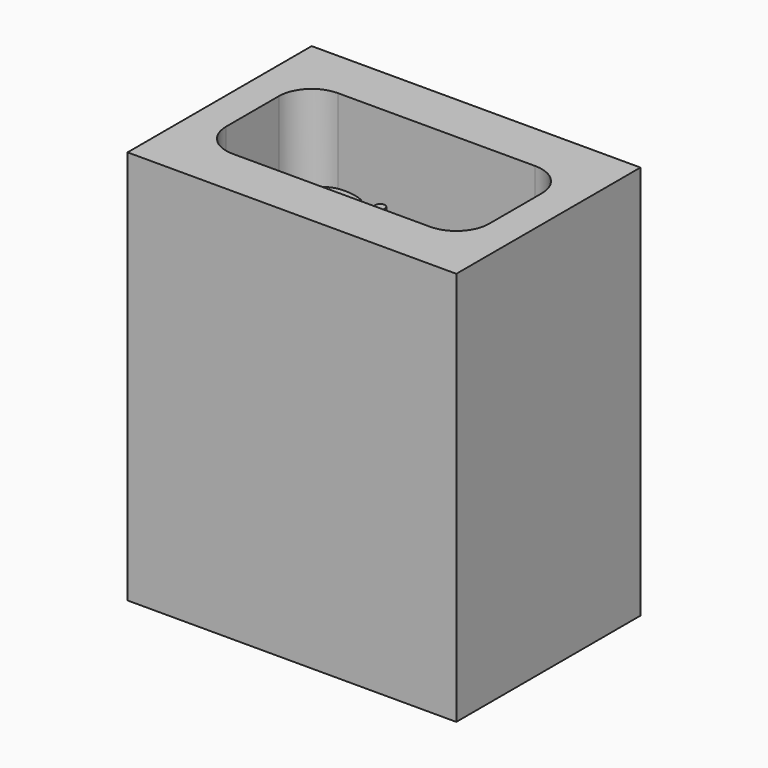
from build123d import *

# Parameters (mm, degrees)
F0_W         = 1000
F0_H         = 700
F1_DEPTH     = 1200
F3_DEPTH     = 300
F4_TEXT_SIZE = 300.7989973367
F5_DEPTH     = 100


# Not quite as in the source:
# - Text() gives the source's letters only with a copy of the font that has no kerning and outlines rounded to 1/6400 em; it was checked with that copy


with BuildPart() as f1:
    # F0 (on Top) → F1 (new body)
    with BuildSketch(Plane.XY):
        Rectangle(F0_W, F0_H)
    extrude(amount=F1_DEPTH)

    # F2 (on face) → F3 (cut)
    with BuildSketch(Plane.XY.offset(1200)):
        with BuildLine():
            Line((-300, -200), (300, -200))
            ThreePointArc((300, -200), (370.7106781187, -170.7106781187), (400, -100))
            Line((400, -100), (400, 100))
            ThreePointArc((400, 100), (370.7106781187, 170.7106781187), (300, 200))
            Line((300, 200), (-300, 200))
            ThreePointArc((-300, 200), (-370.7106781187, 170.7106781187), (-400, 100))
            Line((-400, 100), (-400, -100))
            ThreePointArc((-400, -100), (-370.7106781187, -170.7106781187), (-300, -200))
        make_face()
    extrude(amount=-F3_DEPTH, mode=Mode.SUBTRACT)

    # F4 (on face) → F5 (join)
    with BuildSketch(Plane.XY.offset(900)):
        with Locations((-300, -100)):
            Text('Sink', F4_TEXT_SIZE, font='Open Sans', text_align=(TextAlign.LEFT, TextAlign.BOTTOM))
    extrude(amount=F5_DEPTH)


solid = f1.part
